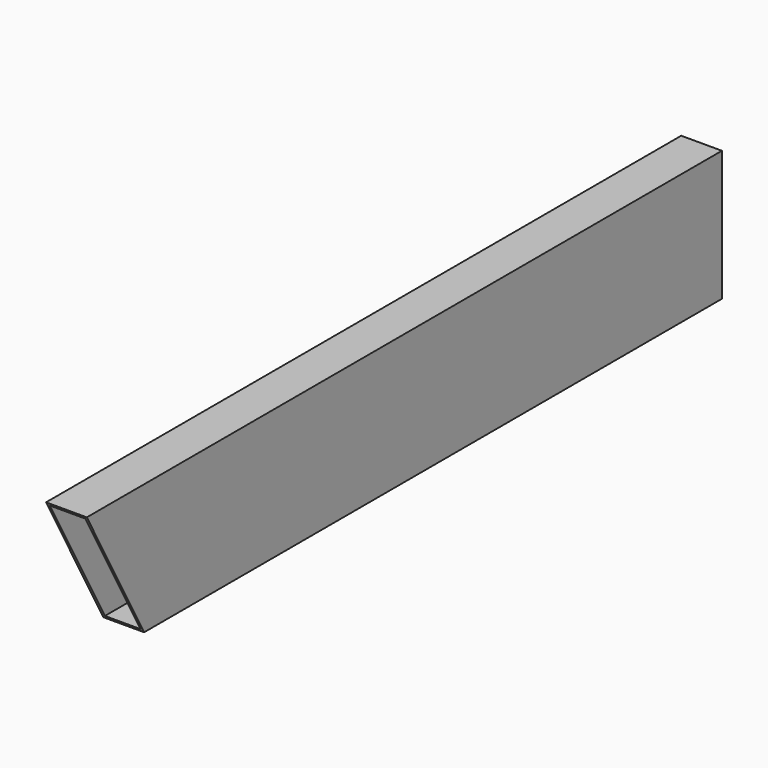
from build123d import *

# Parameters (mm, degrees)
F0_W        = 25
F0_H        = 80
F0_W_2      = 21.83
F0_H_2      = 76.83
F1_DEPTH    = 243.645
F2_T1_DEPTH = 439.0919651514


# Not quite as in the source:
# - a fillet or chamfer that OpenCascade refuses, or shapes differently, is made with other operations: its cross-section is extruded or revolved along the edge and cut away or added


with BuildPart() as f1:
    # F0 (on Front) → F1 (new body, symmetric)
    with BuildSketch(Plane.XZ):
        Rectangle(F0_W, F0_H)
        Rectangle(F0_W_2, F0_H_2, mode=Mode.SUBTRACT)
    extrude(amount=F1_DEPTH, both=True)

    # F2: chamfer of 80 x 43.99 on 1 edges, made by hand

    # F2_s2 → F2_t1 (cut)
    with BuildSketch(Plane.YZ.offset(-219.5459825757)):
        Polygon((-243.645, 40), (-199.655, -40), (-243.645, -40), align=None)
    extrude(amount=F2_T1_DEPTH, mode=Mode.SUBTRACT)


solid = f1.part
